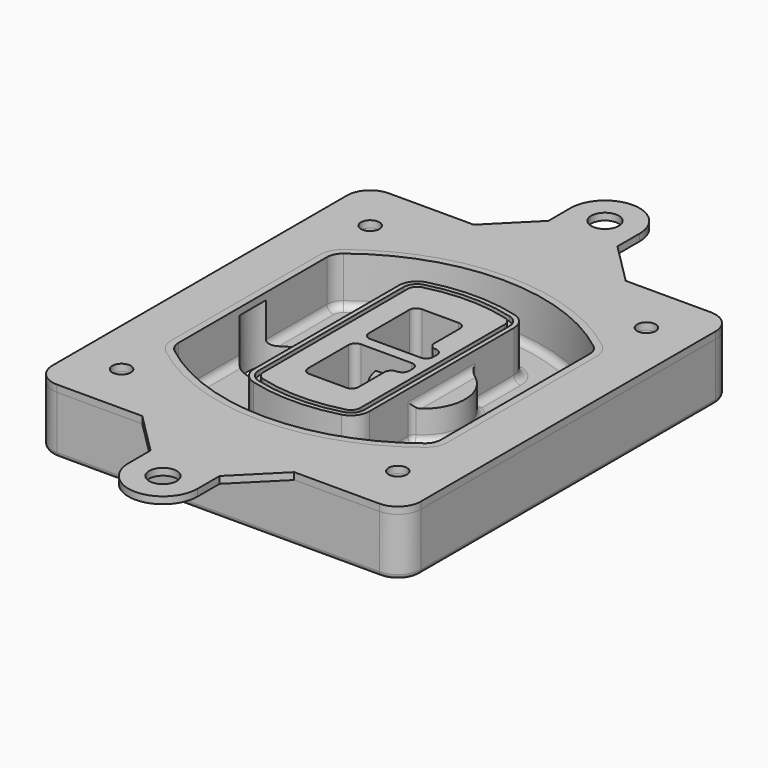
from build123d import *

# Parameters (mm, degrees)
F0_R      = 4
F1_DEPTH  = 25
F2_DEPTH  = 3
F3_DEPTH  = 18
F5_DEPTH  = 21
F6_DEPTH  = 2
F8_DEPTH  = 20
F9_DEPTH  = 16
F10_DEPTH = 25
F7_R      = 6
F7_R_2    = 4
F11_DEPTH = 6
F13_DEPTH = 9
F14_R     = 3
F15_R     = 2
F16_R     = 6
F16_R_2   = 4
F18_DEPTH = 3


# Not quite as in the source:
# - a feature names something its author has since deleted; it is built from what else it names


with BuildPart() as f1:
    # F0 (on Top) → F1 (new body)
    with BuildSketch(Plane.XY):
        with BuildLine():
            ThreePointArc((-80, -80), (-77.0710678119, -87.0710678119), (-70, -90))
            Line((-70, -90), (70, -90))
            ThreePointArc((70, -90), (77.0710678119, -87.0710678119), (80, -80))
            Line((80, -80), (80, 80))
            ThreePointArc((80, 80), (77.0710678119, 87.0710678119), (70, 90))
            Line((70, 90), (-70, 90))
            ThreePointArc((-70, 90), (-77.0710678119, 87.0710678119), (-80, 80))
            Line((-80, 80), (-80, -80))
        make_face()
        with Locations((-60, -67.5)):
            Circle(F0_R, mode=Mode.SUBTRACT)
        with Locations((60, -67.5)):
            Circle(F0_R, mode=Mode.SUBTRACT)
        with Locations((-60, 67.5)):
            Circle(F0_R, mode=Mode.SUBTRACT)
        with BuildLine():
            ThreePointArc((-64, 40.2934422872), (-62.5820384798, 46.4328484224), (-58.6153846154, 51.3286200352))
            ThreePointArc((-58.6153846154, 51.3286200352), (0, 71.5), (58.6153846154, 51.3286200352))
            ThreePointArc((58.6153846154, 51.3286200352), (62.5820384798, 46.4328484224), (64, 40.2934422872))
            Line((64, 40.2934422872), (64, -40.2934422872))
            ThreePointArc((64, -40.2934422872), (62.5820384798, -46.4328484224), (58.6153846154, -51.3286200352))
            ThreePointArc((58.6153846154, -51.3286200352), (0, -71.5), (-58.6153846154, -51.3286200352))
            ThreePointArc((-58.6153846154, -51.3286200352), (-62.5820384798, -46.4328484224), (-64, -40.2934422872))
            Line((-64, -40.2934422872), (-64, 40.2934422872))
        make_face(mode=Mode.SUBTRACT)
        with Locations((60, 67.5)):
            Circle(F0_R, mode=Mode.SUBTRACT)
        with BuildLine():
            ThreePointArc((58.6153846154, 51.3286200352), (0, 71.5), (-58.6153846154, 51.3286200352))
            ThreePointArc((-58.6153846154, 51.3286200352), (-62.5820384798, 46.4328484224), (-64, 40.2934422872))
            Line((-64, 40.2934422872), (-64, -40.2934422872))
            ThreePointArc((-64, -40.2934422872), (-62.5820384798, -46.4328484224), (-58.6153846154, -51.3286200352))
            ThreePointArc((-58.6153846154, -51.3286200352), (0, -71.5), (58.6153846154, -51.3286200352))
            ThreePointArc((58.6153846154, -51.3286200352), (62.5820384798, -46.4328484224), (64, -40.2934422872))
            Line((64, -40.2934422872), (64, 40.2934422872))
            ThreePointArc((64, 40.2934422872), (62.5820384798, 46.4328484224), (58.6153846154, 51.3286200352))
        make_face()
        with BuildLine():
            Line((-60, -40.2934422872), (-60, 40.2934422872))
            ThreePointArc((-60, 40.2934422872), (-58.9871703427, 44.6787323838), (-56.1538461538, 48.1757121072))
            ThreePointArc((-56.1538461538, 48.1757121072), (0, 67.5), (56.1538461538, 48.1757121072))
            ThreePointArc((56.1538461538, 48.1757121072), (58.9871703427, 44.6787323838), (60, 40.2934422872))
            Line((60, 40.2934422872), (60, -40.2934422872))
            ThreePointArc((60, -40.2934422872), (58.9871703427, -44.6787323838), (56.1538461538, -48.1757121072))
            ThreePointArc((56.1538461538, -48.1757121072), (0, -67.5), (-56.1538461538, -48.1757121072))
            ThreePointArc((-56.1538461538, -48.1757121072), (-58.9871703427, -44.6787323838), (-60, -40.2934422872))
        make_face(mode=Mode.SUBTRACT)
        with BuildLine():
            ThreePointArc((-56.1538461538, 48.1757121072), (-58.9871703427, 44.6787323838), (-60, 40.2934422872))
            Line((-60, 40.2934422872), (-60, -40.2934422872))
            ThreePointArc((-60, -40.2934422872), (-58.9871703427, -44.6787323838), (-56.1538461538, -48.1757121072))
            ThreePointArc((-56.1538461538, -48.1757121072), (0, -67.5), (56.1538461538, -48.1757121072))
            ThreePointArc((56.1538461538, -48.1757121072), (58.9871703427, -44.6787323838), (60, -40.2934422872))
            Line((60, -40.2934422872), (60, 40.2934422872))
            ThreePointArc((60, 40.2934422872), (58.9871703427, 44.6787323838), (56.1538461538, 48.1757121072))
            ThreePointArc((56.1538461538, 48.1757121072), (0, 67.5), (-56.1538461538, 48.1757121072))
        make_face()
        with BuildLine():
            ThreePointArc((54.3076923077, 45.8110311612), (56.2910192399, 43.3631453548), (57, 40.2934422872))
            Line((57, 40.2934422872), (57, -40.2934422872))
            ThreePointArc((57, -40.2934422872), (56.2910192399, -43.3631453548), (54.3076923077, -45.8110311612))
            ThreePointArc((54.3076923077, -45.8110311612), (0, -64.5), (-54.3076923077, -45.8110311612))
            ThreePointArc((-54.3076923077, -45.8110311612), (-56.2910192399, -43.3631453548), (-57, -40.2934422872))
            Line((-57, -40.2934422872), (-57, 40.2934422872))
            ThreePointArc((-57, 40.2934422872), (-56.2910192399, 43.3631453548), (-54.3076923077, 45.8110311612))
            ThreePointArc((-54.3076923077, 45.8110311612), (0, 64.5), (54.3076923077, 45.8110311612))
        make_face(mode=Mode.SUBTRACT)
        with BuildLine():
            Line((57, -40.2934422872), (57, 40.2934422872))
            ThreePointArc((57, 40.2934422872), (56.2910192399, 43.3631453548), (54.3076923077, 45.8110311612))
            ThreePointArc((54.3076923077, 45.8110311612), (0, 64.5), (-54.3076923077, 45.8110311612))
            ThreePointArc((-54.3076923077, 45.8110311612), (-56.2910192399, 43.3631453548), (-57, 40.2934422872))
            Line((-57, 40.2934422872), (-57, -40.2934422872))
            ThreePointArc((-57, -40.2934422872), (-56.2910192399, -43.3631453548), (-54.3076923077, -45.8110311612))
            ThreePointArc((-54.3076923077, -45.8110311612), (0, -64.5), (54.3076923077, -45.8110311612))
            ThreePointArc((54.3076923077, -45.8110311612), (56.2910192399, -43.3631453548), (57, -40.2934422872))
        make_face()
    extrude(amount=-F1_DEPTH)

    # F0 (on Top) → F2 (join)
    with BuildSketch(Plane.XY):
        with BuildLine():
            ThreePointArc((-56.1538461538, 48.1757121072), (-58.9871703427, 44.6787323838), (-60, 40.2934422872))
            Line((-60, 40.2934422872), (-60, -40.2934422872))
            ThreePointArc((-60, -40.2934422872), (-58.9871703427, -44.6787323838), (-56.1538461538, -48.1757121072))
            ThreePointArc((-56.1538461538, -48.1757121072), (0, -67.5), (56.1538461538, -48.1757121072))
            ThreePointArc((56.1538461538, -48.1757121072), (58.9871703427, -44.6787323838), (60, -40.2934422872))
            Line((60, -40.2934422872), (60, 40.2934422872))
            ThreePointArc((60, 40.2934422872), (58.9871703427, 44.6787323838), (56.1538461538, 48.1757121072))
            ThreePointArc((56.1538461538, 48.1757121072), (0, 67.5), (-56.1538461538, 48.1757121072))
        make_face()
        with BuildLine():
            ThreePointArc((54.3076923077, 45.8110311612), (56.2910192399, 43.3631453548), (57, 40.2934422872))
            Line((57, 40.2934422872), (57, -40.2934422872))
            ThreePointArc((57, -40.2934422872), (56.2910192399, -43.3631453548), (54.3076923077, -45.8110311612))
            ThreePointArc((54.3076923077, -45.8110311612), (0, -64.5), (-54.3076923077, -45.8110311612))
            ThreePointArc((-54.3076923077, -45.8110311612), (-56.2910192399, -43.3631453548), (-57, -40.2934422872))
            Line((-57, -40.2934422872), (-57, 40.2934422872))
            ThreePointArc((-57, 40.2934422872), (-56.2910192399, 43.3631453548), (-54.3076923077, 45.8110311612))
            ThreePointArc((-54.3076923077, 45.8110311612), (0, 64.5), (54.3076923077, 45.8110311612))
        make_face(mode=Mode.SUBTRACT)
    extrude(amount=F2_DEPTH)

    # F0 (on Top) → F3 (cut)
    with BuildSketch(Plane.XY):
        with BuildLine():
            Line((57, -40.2934422872), (57, 40.2934422872))
            ThreePointArc((57, 40.2934422872), (56.2910192399, 43.3631453548), (54.3076923077, 45.8110311612))
            ThreePointArc((54.3076923077, 45.8110311612), (0, 64.5), (-54.3076923077, 45.8110311612))
            ThreePointArc((-54.3076923077, 45.8110311612), (-56.2910192399, 43.3631453548), (-57, 40.2934422872))
            Line((-57, 40.2934422872), (-57, -40.2934422872))
            ThreePointArc((-57, -40.2934422872), (-56.2910192399, -43.3631453548), (-54.3076923077, -45.8110311612))
            ThreePointArc((-54.3076923077, -45.8110311612), (0, -64.5), (54.3076923077, -45.8110311612))
            ThreePointArc((54.3076923077, -45.8110311612), (56.2910192399, -43.3631453548), (57, -40.2934422872))
        make_face()
    extrude(amount=-F3_DEPTH, mode=Mode.SUBTRACT)

    # F4 (on face) → F5 (join, through all)
    with BuildSketch(Plane.XY.offset(3)):
        with BuildLine():
            ThreePointArc((-25, -39.2465276821), (-23.3511545998, -44.1109737193), (-19.0842911877, -46.9702398883))
            ThreePointArc((-19.0842911877, -46.9702398883), (0, -49.5), (19.0842911877, -46.9702398883))
            ThreePointArc((19.0842911877, -46.9702398883), (23.3511545998, -44.1109737193), (25, -39.2465276821))
            Line((25, -39.2465276821), (25, 39.2465276821))
            ThreePointArc((25, 39.2465276821), (23.3511545998, 44.1109737193), (19.0842911877, 46.9702398883))
            ThreePointArc((19.0842911877, 46.9702398883), (0, 49.5), (-19.0842911877, 46.9702398883))
            ThreePointArc((-19.0842911877, 46.9702398883), (-23.3511545998, 44.1109737193), (-25, 39.2465276821))
            Line((-25, 39.2465276821), (-25, -39.2465276821))
        make_face()
        with BuildLine():
            ThreePointArc((18.5632183908, 45.0393118368), (21.7633659499, 42.89486221), (23, 39.2465276821))
            Line((23, 39.2465276821), (23, -39.2465276821))
            ThreePointArc((23, -39.2465276821), (21.7633659499, -42.89486221), (18.5632183908, -45.0393118368))
            ThreePointArc((18.5632183908, -45.0393118368), (0, -47.5), (-18.5632183908, -45.0393118368))
            ThreePointArc((-18.5632183908, -45.0393118368), (-21.7633659499, -42.89486221), (-23, -39.2465276821))
            Line((-23, -39.2465276821), (-23, 39.2465276821))
            ThreePointArc((-23, 39.2465276821), (-21.7633659499, 42.89486221), (-18.5632183908, 45.0393118368))
            ThreePointArc((-18.5632183908, 45.0393118368), (0, 47.5), (18.5632183908, 45.0393118368))
        make_face(mode=Mode.SUBTRACT)
        with BuildLine():
            Line((23, -39.2465276821), (23, 39.2465276821))
            ThreePointArc((23, 39.2465276821), (21.7633659499, 42.89486221), (18.5632183908, 45.0393118368))
            ThreePointArc((18.5632183908, 45.0393118368), (0, 47.5), (-18.5632183908, 45.0393118368))
            ThreePointArc((-18.5632183908, 45.0393118368), (-21.7633659499, 42.89486221), (-23, 39.2465276821))
            Line((-23, 39.2465276821), (-23, -39.2465276821))
            ThreePointArc((-23, -39.2465276821), (-21.7633659499, -42.89486221), (-18.5632183908, -45.0393118368))
            ThreePointArc((-18.5632183908, -45.0393118368), (0, -47.5), (18.5632183908, -45.0393118368))
            ThreePointArc((18.5632183908, -45.0393118368), (21.7633659499, -42.89486221), (23, -39.2465276821))
        make_face()
        with BuildLine():
            ThreePointArc((18.0421455939, 43.1083837852), (20.1755772999, 41.6787507007), (21, 39.2465276821))
            Line((21, 39.2465276821), (21, -39.2465276821))
            ThreePointArc((21, -39.2465276821), (20.1755772999, -41.6787507007), (18.0421455939, -43.1083837852))
            ThreePointArc((18.0421455939, -43.1083837852), (0, -45.5), (-18.0421455939, -43.1083837852))
            ThreePointArc((-18.0421455939, -43.1083837852), (-20.1755772999, -41.6787507007), (-21, -39.2465276821))
            Line((-21, -39.2465276821), (-21, 39.2465276821))
            ThreePointArc((-21, 39.2465276821), (-20.1755772999, 41.6787507007), (-18.0421455939, 43.1083837852))
            ThreePointArc((-18.0421455939, 43.1083837852), (0, 45.5), (18.0421455939, 43.1083837852))
        make_face(mode=Mode.SUBTRACT)
        with BuildLine():
            Line((21, -39.2465276821), (21, 39.2465276821))
            ThreePointArc((21, 39.2465276821), (20.1755772999, 41.6787507007), (18.0421455939, 43.1083837852))
            ThreePointArc((18.0421455939, 43.1083837852), (0, 45.5), (-18.0421455939, 43.1083837852))
            ThreePointArc((-18.0421455939, 43.1083837852), (-20.1755772999, 41.6787507007), (-21, 39.2465276821))
            Line((-21, 39.2465276821), (-21, -39.2465276821))
            ThreePointArc((-21, -39.2465276821), (-20.1755772999, -41.6787507007), (-18.0421455939, -43.1083837852))
            ThreePointArc((-18.0421455939, -43.1083837852), (0, -45.5), (18.0421455939, -43.1083837852))
            ThreePointArc((18.0421455939, -43.1083837852), (20.1755772999, -41.6787507007), (21, -39.2465276821))
        make_face()
        with BuildLine():
            Line((-8, -2.5), (14, -2.5))
            ThreePointArc((14, -2.5), (16.1213203436, -3.3786796564), (17, -5.5))
            Line((17, -5.5), (17, -7.5))
            ThreePointArc((17, -7.5), (16.1213203436, -9.6213203436), (14, -10.5))
            ThreePointArc((14, -10.5), (11.8786796564, -11.3786796564), (11, -13.5))
            Line((11, -13.5), (11, -27.5))
            ThreePointArc((11, -27.5), (10.1213203436, -29.6213203436), (8, -30.5))
            Line((8, -30.5), (-8, -30.5))
            ThreePointArc((-8, -30.5), (-10.1213203436, -29.6213203436), (-11, -27.5))
            Line((-11, -27.5), (-11, -5.5))
            ThreePointArc((-11, -5.5), (-10.1213203436, -3.3786796564), (-8, -2.5))
        make_face(mode=Mode.SUBTRACT)
        with BuildLine():
            ThreePointArc((-8, 2.5), (-10.1213203436, 3.3786796564), (-11, 5.5))
            Line((-11, 5.5), (-11, 27.5))
            ThreePointArc((-11, 27.5), (-10.1213203436, 29.6213203436), (-8, 30.5))
            Line((-8, 30.5), (8, 30.5))
            ThreePointArc((8, 30.5), (10.1213203436, 29.6213203436), (11, 27.5))
            Line((11, 27.5), (11, 13.5))
            ThreePointArc((11, 13.5), (11.8786796564, 11.3786796564), (14, 10.5))
            ThreePointArc((14, 10.5), (16.1213203436, 9.6213203436), (17, 7.5))
            Line((17, 7.5), (17, 5.5))
            ThreePointArc((17, 5.5), (16.1213203436, 3.3786796564), (14, 2.5))
            Line((14, 2.5), (-8, 2.5))
        make_face(mode=Mode.SUBTRACT)
    extrude(amount=-F5_DEPTH)

    # F4 (on face) → F6 (cut)
    with BuildSketch(Plane.XY.offset(3)):
        with BuildLine():
            Line((23, -39.2465276821), (23, 39.2465276821))
            ThreePointArc((23, 39.2465276821), (21.7633659499, 42.89486221), (18.5632183908, 45.0393118368))
            ThreePointArc((18.5632183908, 45.0393118368), (0, 47.5), (-18.5632183908, 45.0393118368))
            ThreePointArc((-18.5632183908, 45.0393118368), (-21.7633659499, 42.89486221), (-23, 39.2465276821))
            Line((-23, 39.2465276821), (-23, -39.2465276821))
            ThreePointArc((-23, -39.2465276821), (-21.7633659499, -42.89486221), (-18.5632183908, -45.0393118368))
            ThreePointArc((-18.5632183908, -45.0393118368), (0, -47.5), (18.5632183908, -45.0393118368))
            ThreePointArc((18.5632183908, -45.0393118368), (21.7633659499, -42.89486221), (23, -39.2465276821))
        make_face()
        with BuildLine():
            ThreePointArc((18.0421455939, 43.1083837852), (20.1755772999, 41.6787507007), (21, 39.2465276821))
            Line((21, 39.2465276821), (21, -39.2465276821))
            ThreePointArc((21, -39.2465276821), (20.1755772999, -41.6787507007), (18.0421455939, -43.1083837852))
            ThreePointArc((18.0421455939, -43.1083837852), (0, -45.5), (-18.0421455939, -43.1083837852))
            ThreePointArc((-18.0421455939, -43.1083837852), (-20.1755772999, -41.6787507007), (-21, -39.2465276821))
            Line((-21, -39.2465276821), (-21, 39.2465276821))
            ThreePointArc((-21, 39.2465276821), (-20.1755772999, 41.6787507007), (-18.0421455939, 43.1083837852))
            ThreePointArc((-18.0421455939, 43.1083837852), (0, 45.5), (18.0421455939, 43.1083837852))
        make_face(mode=Mode.SUBTRACT)
    extrude(amount=-F6_DEPTH, mode=Mode.SUBTRACT)

    # F7 (on face) → F8 (join)
    with BuildSketch(Plane(origin=(0, 0, -25), x_dir=(1, 0, 0), z_dir=(0, 0, -1))):
        with BuildLine():
            ThreePointArc((3.28842436, 0), (16.7567035675, 13.4682792075), (30.224982775, 0))
            Line((30.224982775, 0), (35.224982775, 0))
            ThreePointArc((35.224982775, 0), (16.7567035675, 18.4682792075), (-1.71157564, 0))
            Line((-1.71157564, 0), (3.28842436, 0))
        make_face()
        with BuildLine():
            Line((3.28842436, 0), (30.224982775, 0))
            ThreePointArc((30.224982775, 0), (16.7567035675, 13.4682792075), (3.28842436, 0))
        make_face()
        with BuildLine():
            ThreePointArc((3.28842436, 0), (16.7567035675, -13.4682792075), (30.224982775, 0))
            Line((30.224982775, 0), (3.28842436, 0))
        make_face()
        with BuildLine():
            Line((35.224982775, 0), (30.224982775, 0))
            ThreePointArc((30.224982775, 0), (16.7567035675, -13.4682792075), (3.28842436, 0))
            Line((3.28842436, 0), (-1.71157564, 0))
            ThreePointArc((-1.71157564, 0), (16.7567035675, -18.4682792075), (35.224982775, 0))
        make_face()
    extrude(amount=-F8_DEPTH)

    # F7 (on face) → F9 (cut)
    with BuildSketch(Plane(origin=(0, 0, -25), x_dir=(1, 0, 0), z_dir=(0, 0, -1))):
        with BuildLine():
            Line((3.28842436, 0), (30.224982775, 0))
            ThreePointArc((30.224982775, 0), (16.7567035675, 13.4682792075), (3.28842436, 0))
        make_face()
        with BuildLine():
            ThreePointArc((3.28842436, 0), (16.7567035675, -13.4682792075), (30.224982775, 0))
            Line((30.224982775, 0), (3.28842436, 0))
        make_face()
    extrude(amount=-F9_DEPTH, mode=Mode.SUBTRACT)

    # F7 (on face) → F10 (cut)
    with BuildSketch(Plane(origin=(0, 0, -25), x_dir=(1, 0, 0), z_dir=(0, 0, -1))):
        with BuildLine():
            Line((-59.0318229325, 0), (-32.0952645175, 0))
            ThreePointArc((-32.0952645175, 0), (-45.563543725, 13.4682792075), (-59.0318229325, 0))
        make_face()
        with BuildLine():
            ThreePointArc((-59.0318229325, 0), (-45.563543725, -13.4682792075), (-32.0952645175, 0))
            Line((-32.0952645175, 0), (-59.0318229325, 0))
        make_face()
    extrude(amount=-F10_DEPTH, mode=Mode.SUBTRACT)

    # F7 (on face) → F11 (cut)
    with BuildSketch(Plane(origin=(0, 0, -25), x_dir=(1, 0, 0), z_dir=(0, 0, -1))):
        with Locations((60, -67.5)):
            Circle(F7_R)
        with Locations((60, -67.5)):
            Circle(F7_R_2, mode=Mode.SUBTRACT)
        with Locations((-60, -67.5)):
            Circle(F7_R)
        with Locations((-60, -67.5)):
            Circle(F7_R_2, mode=Mode.SUBTRACT)
        with Locations((-60, 67.5)):
            Circle(F7_R)
        with Locations((-60, 67.5)):
            Circle(F7_R_2, mode=Mode.SUBTRACT)
        with Locations((60, 67.5)):
            Circle(F7_R)
        with Locations((60, 67.5)):
            Circle(F7_R_2, mode=Mode.SUBTRACT)
    extrude(amount=-F11_DEPTH, mode=Mode.SUBTRACT)

    # F12 (on face) → F13 (cut, through all)
    with BuildSketch(Plane(origin=(0, 0, -9), x_dir=(1, 0, 0), z_dir=(0, 0, -1))):
        with BuildLine():
            Line((11, 13.5), (11, 17.5481537753))
            ThreePointArc((11, 17.5481537753), (2.5696536419, 11.8239143813), (-1.5415842455, 2.5))
            Line((-1.5415842455, 2.5), (3.5224848595, 2.5))
            ThreePointArc((3.5224848595, 2.5), (6.1857188154, 8.3455872281), (11.2536447004, 12.2927168648))
            ThreePointArc((11.2536447004, 12.2927168648), (11.0640958889, 12.8831798879), (11, 13.5))
        make_face()
        with BuildLine():
            ThreePointArc((11.2536447004, -12.2927168648), (6.1857188154, -8.3455872281), (3.5224848595, -2.5))
            Line((3.5224848595, -2.5), (-1.5415842455, -2.5))
            ThreePointArc((-1.5415842455, -2.5), (2.5696536419, -11.8239143813), (11, -17.5481537753))
            Line((11, -17.5481537753), (11, -13.5))
            ThreePointArc((11, -13.5), (11.0640958889, -12.8831798879), (11.2536447004, -12.2927168648))
        make_face()
        with BuildLine():
            ThreePointArc((11.2536447004, 12.2927168648), (6.1857188154, 8.3455872281), (3.5224848595, 2.5))
            Line((3.5224848595, 2.5), (14, 2.5))
            ThreePointArc((14, 2.5), (16.1213203436, 3.3786796564), (17, 5.5))
            Line((17, 5.5), (17, 7.5))
            ThreePointArc((17, 7.5), (16.1213203436, 9.6213203436), (14, 10.5))
            ThreePointArc((14, 10.5), (12.3601599782, 10.9878446101), (11.2536447004, 12.2927168648))
        make_face()
        with BuildLine():
            Line((14, -2.5), (3.5224848595, -2.5))
            ThreePointArc((3.5224848595, -2.5), (6.1857188154, -8.3455872281), (11.2536447004, -12.2927168648))
            ThreePointArc((11.2536447004, -12.2927168648), (12.3601599782, -10.9878446101), (14, -10.5))
            ThreePointArc((14, -10.5), (16.1213203436, -9.6213203436), (17, -7.5))
            Line((17, -7.5), (17, -5.5))
            ThreePointArc((17, -5.5), (16.1213203436, -3.3786796564), (14, -2.5))
        make_face()
    extrude(amount=F13_DEPTH, mode=Mode.SUBTRACT)

    # F14
    f14_edges = [f1.edges().sort_by_distance(p)[0] for p in [
        (-57, -23.703476, -18),
        (-57, 23.703476, -18),
        (25, 0, -5),
        (25, 16.526506, -11.5),
        (25, -16.526506, -11.5),
        (25, -27.886517, -18),
        (35.224983, 0, -18),
    ]]
    fillet(f14_edges, radius=F14_R)

    # F15
    f15_edges = [f1.edges().sort_by_distance(p)[0] for p in [
        (0, -90, -25),
    ]]
    fillet(f15_edges, radius=F15_R)


with BuildPart() as f18:
    # F16 (on face) → F18 (new body, through all)
    with BuildSketch(Plane.XY):
        with BuildLine():
            Line((33, -90), (-33, -90))
            Line((-33, -90), (-15, -108))
            Line((-15, -108), (-15, -120))
            ThreePointArc((-15, -120), (0, -135), (15, -120))
            Line((15, -120), (15, -108))
            Line((15, -108), (33, -90))
        make_face()
        with Locations((0, -120)):
            Circle(F16_R, mode=Mode.SUBTRACT)
        with BuildLine():
            Line((-15, 108), (-33, 90))
            Line((-33, 90), (33, 90))
            Line((33, 90), (15, 108))
            Line((15, 108), (15, 120))
            ThreePointArc((15, 120), (0, 135), (-15, 120))
            Line((-15, 120), (-15, 108))
        make_face()
        with Locations((0, 120)):
            Circle(F16_R, mode=Mode.SUBTRACT)
        with BuildLine():
            Line((33, 90), (-33, 90))
            Line((-33, 90), (-70, 90))
            ThreePointArc((-70, 90), (-77.0710678119, 87.0710678119), (-80, 80))
            Line((-80, 80), (-80, -80))
            ThreePointArc((-80, -80), (-77.0710678119, -87.0710678119), (-70, -90))
            Line((-70, -90), (-33, -90))
            Line((-33, -90), (33, -90))
            Line((33, -90), (70, -90))
            ThreePointArc((70, -90), (77.0710678119, -87.0710678119), (80, -80))
            Line((80, -80), (80, 80))
            ThreePointArc((80, 80), (77.0710678119, 87.0710678119), (70, 90))
            Line((70, 90), (33, 90))
        make_face()
        with Locations((-60, -67.5)):
            Circle(F16_R_2, mode=Mode.SUBTRACT)
        with Locations((60, -67.5)):
            Circle(F16_R_2, mode=Mode.SUBTRACT)
        with Locations((-60, 67.5)):
            Circle(F16_R_2, mode=Mode.SUBTRACT)
        with BuildLine():
            ThreePointArc((-60, 40.2934422872), (-58.9871703427, 44.6787323838), (-56.1538461538, 48.1757121072))
            ThreePointArc((-56.1538461538, 48.1757121072), (0, 67.5), (56.1538461538, 48.1757121072))
            ThreePointArc((56.1538461538, 48.1757121072), (58.9871703427, 44.6787323838), (60, 40.2934422872))
            Line((60, 40.2934422872), (60, -40.2934422872))
            ThreePointArc((60, -40.2934422872), (58.9871703427, -44.6787323838), (56.1538461538, -48.1757121072))
            ThreePointArc((56.1538461538, -48.1757121072), (0, -67.5), (-56.1538461538, -48.1757121072))
            ThreePointArc((-56.1538461538, -48.1757121072), (-58.9871703427, -44.6787323838), (-60, -40.2934422872))
            Line((-60, -40.2934422872), (-60, 40.2934422872))
        make_face(mode=Mode.SUBTRACT)
        with Locations((60, 67.5)):
            Circle(F16_R_2, mode=Mode.SUBTRACT)
    extrude(amount=F18_DEPTH)


solid = Compound([f1.part, f18.part])
